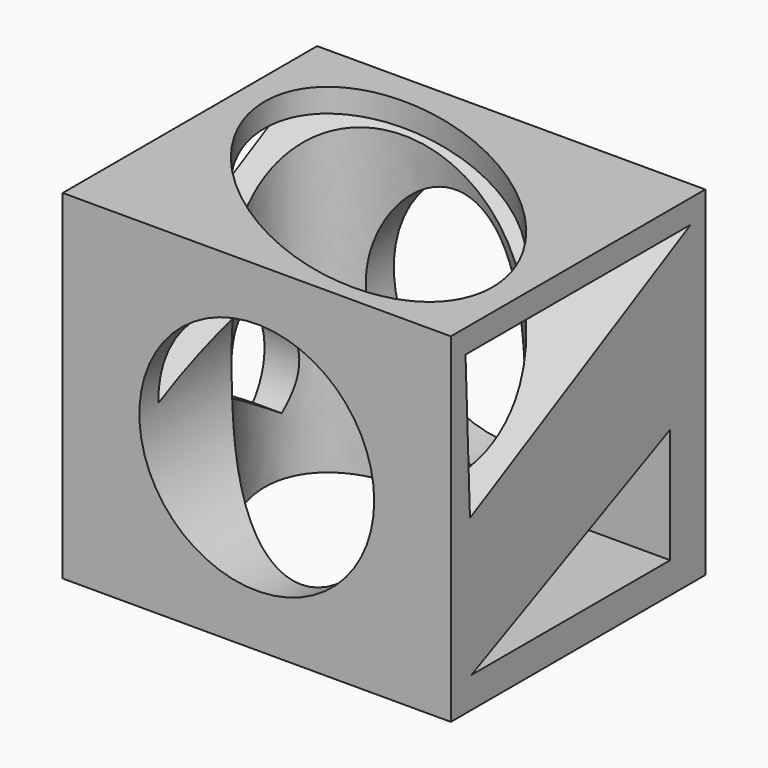
from build123d import *

# Parameters (mm, degrees)
F0_W      = 61.9896091521
F0_H      = 54.219648242
F1_DEPTH  = 50.8
F2_R      = 18.7550893508
F3_DEPTH  = 50.8
F5_DEPTH  = 76.2
F7_DEPTH  = 25.4
F9_DEPTH  = 25.4
F11_DEPTH = 76.2


# Not quite as in the source:
# - the program builds the solid bodies; features that only make, move or delete a surface that nothing else refers to are left out


with BuildPart() as f1:
    # F0 (on Front) → F1 (new body)
    with BuildSketch(Plane.XZ):
        Rectangle(F0_W, F0_H)
    extrude(amount=F1_DEPTH)

    # F2 (on face) → F3 (cut)
    with BuildSketch(Plane.XZ.offset(50.8)):
        Circle(F2_R)
    extrude(amount=-F3_DEPTH, mode=Mode.SUBTRACT)

    # F4 (on face) → F5 (cut)
    with BuildSketch(Plane.YZ.offset(30.994804576)):
        Polygon((-2.9180375859, 23.3443211764), (-47.8669425896, 23.3443211764), (-46.9804480672, 0), align=None)
    extrude(amount=-F5_DEPTH, mode=Mode.SUBTRACT)

    # F6 (on face) → F7 (cut)
    with BuildSketch(Plane.YZ.offset(30.994804576)):
        Polygon((-7.0032961667, -3.7934524007), (-46.6886423528, -22.1771057695), (-7.0032961667, -22.1771057695), align=None)
    extrude(amount=-F7_DEPTH, mode=Mode.SUBTRACT)

    # F8 (on face) → F9 (cut)
    with BuildSketch(Plane(origin=(-30.994804576, 0, 0), x_dir=(0, -1, 0), z_dir=(-1, 0, 0))):
        with BuildLine():
            ThreePointArc((31.5148383379, -6.0229151244), (27.3993926797, -1.8933707931), (21.8853037804, 0))
            ThreePointArc((21.8853037804, 0), (11.700935396, -6.0229151244), (12.8393778577, -17.800046131))
            Line((12.8393778577, -17.800046131), (31.5148383379, -6.0229151244))
        make_face()
    extrude(amount=-F9_DEPTH, mode=Mode.SUBTRACT)

    # F10 (on face) → F11 (cut)
    with BuildSketch(Plane(origin=(0, 0, -27.109824121), x_dir=(1, 0, 0), z_dir=(0, 0, -1))):
        with BuildLine():
            add(Edge.make_bspline(
                [(25.1382775605, 42.9783463478), (9.257748975, 67.1896429686), (-20.509403073, 30.3511721059), (-50.2765551209, -6.4872987568), (-4.6288744875, 6.1398754851), (41.018806146, 18.767049727), (25.1382775605, 42.9783463478)],
                knots=[0, 0, 0, 2.0943951024, 2.0943951024, 4.1887902048, 4.1887902048, 6.2831853072, 6.2831853072, 6.2831853072], degree=2, weights=[1, 0.5, 1, 0.5, 1, 0.5, 1]))
        make_face()
    extrude(amount=-F11_DEPTH, mode=Mode.SUBTRACT)


solid = f1.part
